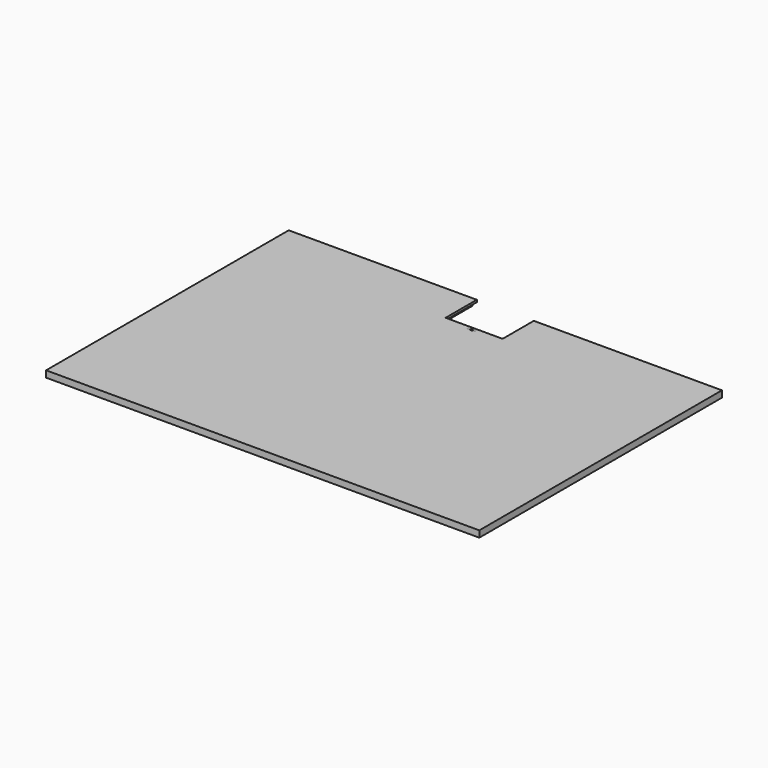
from build123d import *

# Parameters (mm, degrees)
F0_W      = 2000
F0_H      = 1400
F1_DEPTH  = 30
F3_DEPTH  = 180
F4_R      = 6
F5_DEPTH  = 20
F6_W      = 40
F6_H      = 10
F7_DEPTH  = 2
F9_W      = 37
F9_H      = 7
F10_DEPTH = 28.001
F12_DEPTH = 2
F13_W     = 37
F13_H     = 7
F14_DEPTH = 28
F15_DEPTH = 12.5
F16_DEPTH = 1
F17_R     = 0.3


with BuildPart() as f1:
    # F0 (on Top) → F1 (new body)
    with BuildSketch(Plane.XY):
        Rectangle(F0_W, F0_H)
    extrude(amount=F1_DEPTH)

    # F2 (on face) → F3 (cut)
    with BuildSketch(Plane(origin=(0, 700, 0), x_dir=(-1, 0, 0), z_dir=(0, 1, 0))):
        Polygon((-161.5470053838, 20), (-150, 0), (150, 0), (161.5470053838, 20), (131.5470053838, 20), (131.5470053838, 30), (-131.5470053838, 30), (-131.5470053838, 20), align=None)
    extrude(amount=-F3_DEPTH, mode=Mode.SUBTRACT)

    # F4 (on face) → F5 (cut)
    with BuildSketch(Plane(origin=(0, 520, 0), x_dir=(-1, 0, 0), z_dir=(0, 1, 0))):
        with Locations((0, 15)):
            Circle(F4_R)
    extrude(amount=-F5_DEPTH, mode=Mode.SUBTRACT)

    # F6 (on face) → F7 (cut)
    with BuildSketch(Plane(origin=(0, 0, 0), x_dir=(1, 0, 0), z_dir=(0, 0, -1))):
        with Locations((0, -505)):
            Rectangle(F6_W, F6_H)
    extrude(amount=-F7_DEPTH, mode=Mode.SUBTRACT)

    # F9 (on face) → F10 (cut, through all)
    with BuildSketch(Plane(origin=(0, 0, 2), x_dir=(1, 0, 0), z_dir=(0, 0, -1))):
        with Locations((0, -505)):
            Rectangle(F9_W, F9_H)
    extrude(amount=-F10_DEPTH, mode=Mode.SUBTRACT)


with BuildPart() as f12:
    # F6 (on face) → F12 (new body, through all)
    with BuildSketch(Plane(origin=(0, 0, 0), x_dir=(1, 0, 0), z_dir=(0, 0, -1))):
        with Locations((0, -505)):
            Rectangle(F6_W, F6_H)
    extrude(amount=-F12_DEPTH)

    # F13 (on face) → F14 (join, through all)
    with BuildSketch(Plane.XY.offset(2)):
        with Locations((0, 505)):
            Rectangle(F13_W, F13_H)
    extrude(amount=F14_DEPTH)

    # F11 (on offset) → F15 (cut, symmetric)
    with BuildSketch(Plane(origin=(0, 505, 0), x_dir=(-1, 0, 0), z_dir=(0, 1, 0))):
        with BuildLine():
            ThreePointArc((-6, 15), (0, 21), (6, 15))
            Line((6, 15), (6, 30))
            Line((6, 30), (-6, 30))
            Line((-6, 30), (-6, 15))
        make_face()
        with BuildLine():
            Line((4.5, 15), (6, 15))
            ThreePointArc((6, 15), (0, 21), (-6, 15))
            Line((-6, 15), (-4.5, 15))
            ThreePointArc((-4.5, 15), (0, 19.5), (4.5, 15))
        make_face()
        with BuildLine():
            Line((-4.5, 15), (4.5, 15))
            ThreePointArc((4.5, 15), (0, 19.5), (-4.5, 15))
        make_face()
        with BuildLine():
            ThreePointArc((-4.5, 15), (0, 10.5), (4.5, 15))
            Line((4.5, 15), (-4.5, 15))
        make_face()
        with BuildLine():
            ThreePointArc((-6, 15), (0, 9), (6, 15))
            Line((6, 15), (4.5, 15))
            ThreePointArc((4.5, 15), (0, 10.5), (-4.5, 15))
            Line((-4.5, 15), (-6, 15))
        make_face()
    extrude(amount=F15_DEPTH, both=True, mode=Mode.SUBTRACT)

    # F11 (on offset) → F16 (join, symmetric)
    with BuildSketch(Plane(origin=(0, 505, 0), x_dir=(-1, 0, 0), z_dir=(0, 1, 0))):
        with BuildLine():
            ThreePointArc((-6, 15), (0, 9), (6, 15))
            Line((6, 15), (4.5, 15))
            ThreePointArc((4.5, 15), (0, 10.5), (-4.5, 15))
            Line((-4.5, 15), (-6, 15))
        make_face()
    extrude(amount=F16_DEPTH, both=True)

    # F17
    f17_edges = [f12.edges().sort_by_distance(p)[0] for p in [
        (4.5, 505, 15),
        (5.25, 504, 15),
        (0, 506, 10.5),
        (0, 504, 10.5),
        (5.25, 506, 15),
        (-5.25, 506, 15),
        (-4.5, 505, 15),
        (-5.25, 504, 15),
    ]]
    fillet(f17_edges, radius=F17_R)


solid = Compound([f1.part, f12.part])
